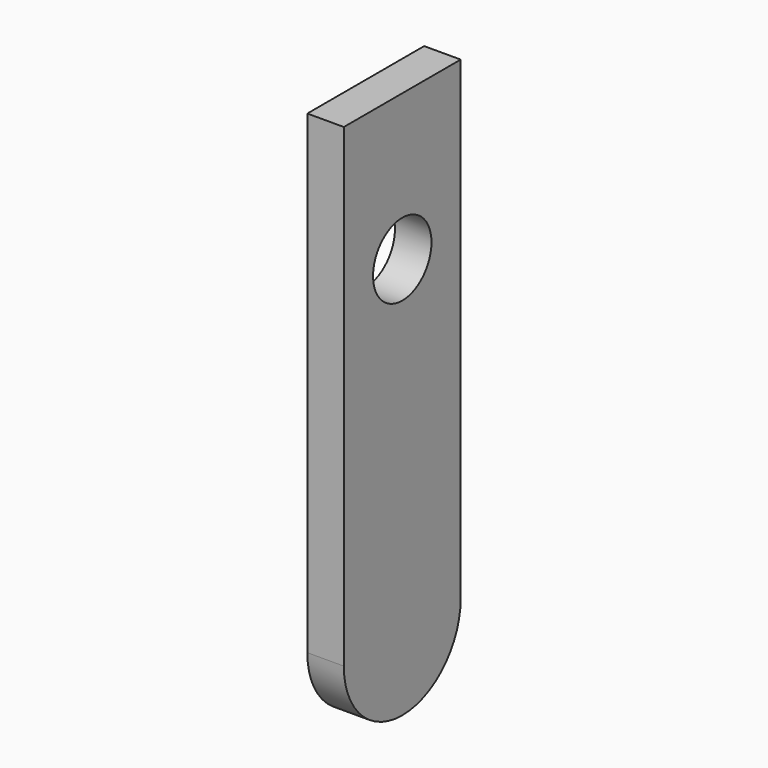
from build123d import *

# Parameters (mm, degrees)
F0_W     = 25.4
F0_H     = 95.25
F0_R     = 6.35
F1_DEPTH = 3.175
F2_R     = 12.69999


# Not quite as in the source:
# - a fillet or chamfer is up to 0.001 mm smaller than in the source, because OpenCascade refuses the exact size


with BuildPart() as f1:
    # F0 (on Right) → F1 (new body, symmetric)
    with BuildSketch(Plane.YZ):
        Rectangle(F0_W, F0_H)
        with Locations((0, 22.225)):
            Circle(F0_R, mode=Mode.SUBTRACT)
    extrude(amount=F1_DEPTH, both=True)

    # F2 (radius 12.7 in the source; OpenCascade refuses exactly that, so slightly less here)
    f2_edges = [f1.edges().sort_by_distance(p)[0] for p in [
        (0, 12.7, -47.625),
        (0, -12.7, -47.625),
    ]]
    fillet(f2_edges, radius=F2_R)


solid = f1.part
